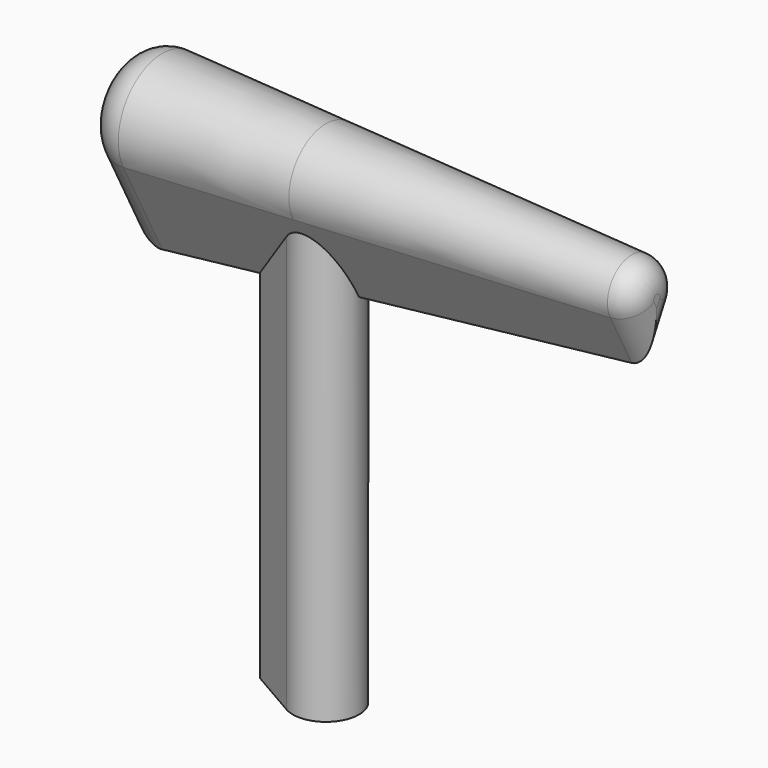
from build123d import *

# Parameters (mm, degrees)
F1_DEPTH               = 177.8
F3_DEPTH               = 127
DRAFT_F3_DRAFTED_ANGLE = 3
F5_DEPTH               = 76.2
DRAFT_F5_DRAFTED_ANGLE = -3
F6_R                   = 10.16
F7_R                   = 12.7


# Not quite as in the source:
# - an extrude with a draft is written as a straight extrude whose walls are then drafted


with BuildPart() as f1:
    # F0 (on Top) → F1 (new body)
    with BuildSketch(Plane.XY):
        with BuildLine():
            Line((-25.4, 0), (-6.35, -10.9985226281))
            ThreePointArc((-6.35, -10.9985226281), (12.7, 0), (-6.35, 10.9985226281))
            Line((-6.35, 10.9985226281), (-25.4, 0))
        make_face()
    extrude(amount=F1_DEPTH)


with BuildPart() as f3_drafted:
    # F2 (on Right) → F3 (new body)
    with BuildSketch(Plane.YZ):
        with BuildLine():
            Line((0, 139.7), (15.7252236727, 169.5026666667))
            ThreePointArc((15.7252236727, 169.5026666667), (0, 195.58), (-15.7252236727, 169.5026666667))
            Line((-15.7252236727, 169.5026666667), (0, 139.7))
        make_face()
    extrude(amount=F3_DEPTH)

    # draft_F3_drafted
    draft_f3_drafted_walls = [f3_drafted.faces().sort_by_distance(p)[0] for p in [
        (84.6666666667, -7.8626118363, 154.6013333333),
        (84.6666666667, 7.8626118363, 154.6013333333),
        (84.6666666667, 0, 195.58),
    ]]
    draft(draft_f3_drafted_walls, neutral_plane=Plane.YZ, angle=DRAFT_F3_DRAFTED_ANGLE)


with BuildPart() as f1_1:
    add(f1.part)

    # join_F3_drafted: union F3_drafted
    add(f3_drafted.part)


with BuildPart() as f5_drafted:
    # F4 (on face) → F5 (new body)
    with BuildSketch(Plane(origin=(0, 0, 0), x_dir=(0, -1, 0), z_dir=(-1, 0, 0))):
        with BuildLine():
            ThreePointArc((15.725223672, 169.5026666653), (1.5e-09, 195.58), (-15.7252236734, 169.502666668))
            Line((-15.7252236759, 169.5026666667), (-3.2e-09, 139.7))
            Line((-3.2e-09, 139.7), (15.7252236695, 169.5026666667))
        make_face()
    extrude(amount=F5_DEPTH)

    # draft_F5_drafted
    draft_f5_drafted_walls = [f5_drafted.faces().sort_by_distance(p)[0] for p in [
        (-50.8, -1.5e-09, 195.58),
        (-50.8, 7.8626118396, 154.6013333333),
        (-50.8, -7.8626118331, 154.6013333333),
    ]]
    draft(draft_f5_drafted_walls, neutral_plane=Plane(origin=(0, 0, 0), x_dir=(0, -1, 0), z_dir=(-1, 0, 0)), angle=DRAFT_F5_DRAFTED_ANGLE)


with BuildPart() as f1_2:
    add(f1_1.part)

    # join_F5_drafted: union F5_drafted
    add(f5_drafted.part)

    # F6
    f6_edges = [f1_2.edges().sort_by_distance(p)[0] for p in [
        (127, 4.919312, 163.285552),
        (127, -4.919312, 163.285552),
        (127, 0, 188.924212),
    ]]
    fillet(f6_edges, radius=F6_R)

    # F7
    f7_edges = [f1_2.edges().sort_by_distance(p)[0] for p in [
        (-76.2, 9.628592, 149.390802),
        (-76.2, -9.628592, 149.390802),
        (-76.2, 0, 199.573473),
    ]]
    fillet(f7_edges, radius=F7_R)


solid = f1_2.part
